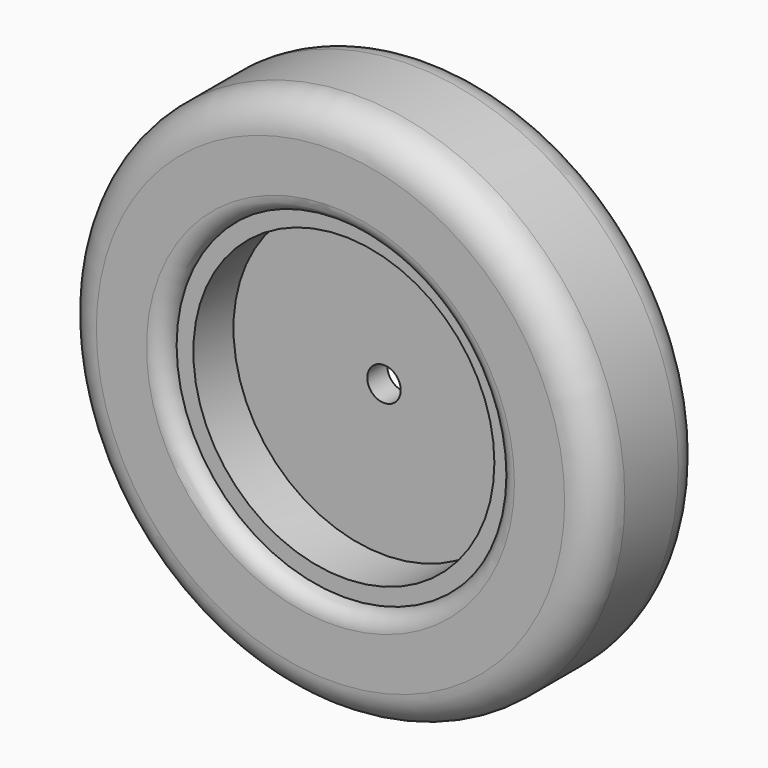
from build123d import *

# Parameters (mm, degrees)
F0_R     = 203.2
F0_R_2   = 127
F1_DEPTH = 50.8
F2_DEPTH = 50.8
F0_R_3   = 114.3
F3_DEPTH = 38.1
F4_DEPTH = 38.1
F5_R     = 25.4
F6_R     = 12.69999
F0_R_4   = 12.7
F7_DEPTH = 19.05


# Not quite as in the source:
# - a fillet or chamfer is up to 0.001 mm smaller than in the source, because OpenCascade refuses the exact size


with BuildPart() as f1:
    # F0 (on Front) → F1 (new body)
    with BuildSketch(Plane.XZ):
        Circle(F0_R)
        Circle(F0_R_2, mode=Mode.SUBTRACT)
    extrude(amount=F1_DEPTH)

    # F0 (on Front) → F2 (join)
    with BuildSketch(Plane.XZ):
        Circle(F0_R)
        Circle(F0_R_2, mode=Mode.SUBTRACT)
    extrude(amount=-F2_DEPTH)

    # F0 (on Front) → F3 (join)
    with BuildSketch(Plane.XZ):
        Circle(F0_R_2)
        Circle(F0_R_3, mode=Mode.SUBTRACT)
    extrude(amount=F3_DEPTH)

    # F0 (on Front) → F4 (join)
    with BuildSketch(Plane.XZ):
        Circle(F0_R_2)
        Circle(F0_R_3, mode=Mode.SUBTRACT)
    extrude(amount=-F4_DEPTH)

    # F5
    f5_edges = [f1.edges().sort_by_distance(p)[0] for p in [
        (-203.2, -50.8, 0),
        (-203.2, 50.8, 0),
    ]]
    fillet(f5_edges, radius=F5_R)

    # F6 (radius 12.7 in the source; OpenCascade refuses exactly that, so slightly less here)
    f6_edges = [f1.edges().sort_by_distance(p)[0] for p in [
        (-127, -50.8, 0),
        (-127, 50.8, 0),
    ]]
    fillet(f6_edges, radius=F6_R)

    # F0 (on Front) → F7 (join)
    with BuildSketch(Plane.XZ):
        Circle(F0_R_3)
        Circle(F0_R_4, mode=Mode.SUBTRACT)
    extrude(amount=-F7_DEPTH)


solid = f1.part
